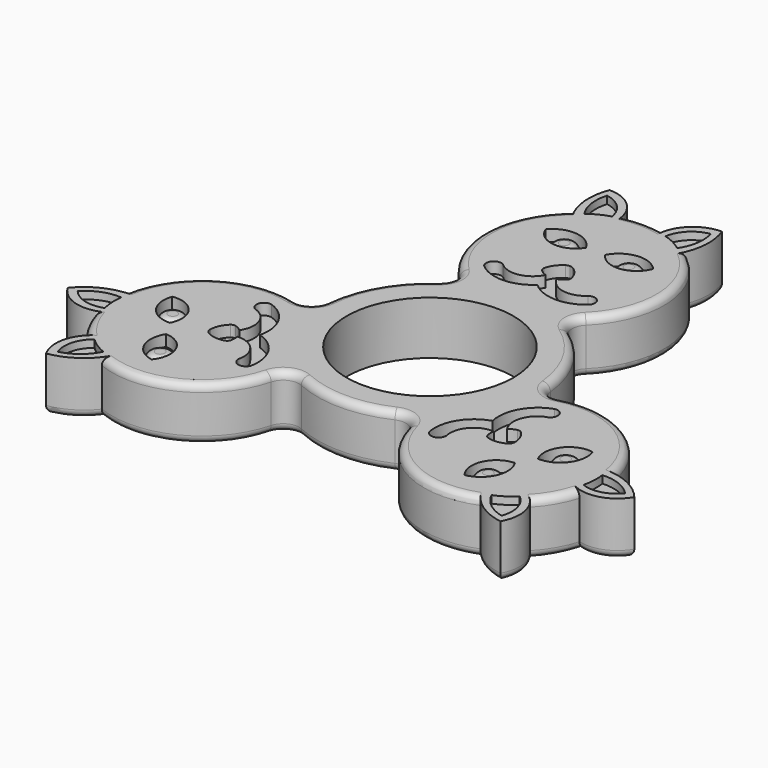
from build123d import *

# Parameters (mm, degrees)
F0_R           = 15
F0_R_2         = 11.125
F1_DEPTH       = 7.1
F3_DEPTH       = 7.1
F5_DEPTH       = 1.5
F6_R           = 1.6130876501
F7_DEPTH       = 1
F8_R           = 0.99999
F10_DEPTH      = 1
F11_R          = 1
F12_T4_ANGLE   = 109.1117538583
F12_S5_R       = 8.0010963912
F12_T6_DEPTH   = 12
F12_T10_ANGLE  = 78.8114219242
F12_S11_R      = 12
F12_T12_DEPTH  = 7
F12_T16_ANGLE  = 134.4694121448
F12_S17_R      = 12
F12_T18_DEPTH  = 7
F12_T22_ANGLE  = 50.774655832
F12_S23_R      = 4.8516880278
F12_T24_DEPTH  = 7
F12_S25_R      = 4.8516880278
F12_T26_DEPTH  = 7
F12_T30_ANGLE  = 134.4694121448
F12_S31_R      = 12
F12_T32_DEPTH  = 7
F12_T36_ANGLE  = 78.8114219242
F12_S37_R      = 12
F12_T38_DEPTH  = 7
F12_T42_ANGLE  = 109.1117538583
F12_S43_R      = 8.0010963912
F12_T44_DEPTH  = 13
F12_T48_ANGLE  = 78.8114219242
F12_S49_R      = 12
F12_T50_DEPTH  = 7
F12_T54_ANGLE  = 134.4694121448
F12_S55_R      = 12
F12_T56_DEPTH  = 7
F12_T60_ANGLE  = 50.774655832
F12_S61_R      = 4.8516880278
F12_T62_DEPTH  = 8
F12_S63_R      = 4.8516880278
F12_T64_DEPTH  = 8
F12_T68_ANGLE  = 134.4694121448
F12_S69_R      = 12
F12_T70_DEPTH  = 7
F12_T74_ANGLE  = 78.8114219242
F12_S75_R      = 12
F12_T76_DEPTH  = 7
F12_T80_ANGLE  = 109.1117538583
F12_S81_R      = 8.0010963912
F12_T82_DEPTH  = 13
F12_T86_ANGLE  = 78.8114219242
F12_S87_R      = 12
F12_T88_DEPTH  = 7
F12_T92_ANGLE  = 134.4694121448
F12_S93_R      = 12
F12_T94_DEPTH  = 7
F12_T98_ANGLE  = 50.774655832
F12_S99_R      = 4.8516880278
F12_T100_DEPTH = 7
F12_S101_R     = 4.8516880278
F12_T102_DEPTH = 7
F12_T106_ANGLE = 134.4694121448
F12_S107_R     = 12
F12_T108_DEPTH = 7
F12_T112_ANGLE = 78.8114219242
F12_S113_R     = 12
F12_T114_DEPTH = 7
F12_T116_ANGLE = 100.004132084
F12_T118_ANGLE = 49.2209251177
F12_T120_ANGLE = 100.004132084
F12_T124_ANGLE = 109.1117538583
F12_S125_R     = 8.0010963912
F12_T126_DEPTH = 13
F12_T128_ANGLE = 100.004132084
F12_T130_ANGLE = 49.2209251177
F12_T132_ANGLE = 100.004132084
F12_T136_ANGLE = 109.1117538583
F12_S137_R     = 8.0010963912
F12_T138_DEPTH = 12
F12_T140_ANGLE = 100.004132084
F12_T142_ANGLE = 49.2209251177
F12_T144_ANGLE = 100.004132084
F12_T148_ANGLE = 109.1117538583
F12_S149_R     = 8.0010963912
F12_T150_DEPTH = 13
F12_T155_ANGLE = 78.8114219242
F12_S156_R     = 12
F12_T157_DEPTH = 7
F12_T160_ANGLE = 109.1117538583
F12_S161_R     = 8.0010963912
F12_T162_DEPTH = 12
F12_T168_ANGLE = 78.8114219242
F12_S169_R     = 12
F12_T170_DEPTH = 7
F12_T173_ANGLE = 109.1117538583
F12_S174_R     = 8.0010963912
F12_T175_DEPTH = 13
F12_T181_ANGLE = 134.4694121448
F12_S182_R     = 12
F12_T183_DEPTH = 7
F12_T186_ANGLE = 50.774655832
F12_S187_R     = 4.8516880278
F12_T188_DEPTH = 7
F12_T194_ANGLE = 134.4694121448
F12_S195_R     = 12
F12_T196_DEPTH = 7
F12_T199_ANGLE = 50.774655832
F12_S200_R     = 4.8516880278
F12_T201_DEPTH = 7
F12_T207_ANGLE = 78.8114219242
F12_S208_R     = 12
F12_T209_DEPTH = 7
F12_T212_ANGLE = 109.1117538583
F12_S213_R     = 8.0010963912
F12_T214_DEPTH = 13
F12_T220_ANGLE = 78.8114219242
F12_S221_R     = 12
F12_T222_DEPTH = 7
F12_T225_ANGLE = 109.1117538583
F12_S226_R     = 8.0010963912
F12_T227_DEPTH = 12
F12_T233_ANGLE = 134.4694121448
F12_S234_R     = 12
F12_T235_DEPTH = 7
F12_T238_ANGLE = 50.774655832
F12_S239_R     = 4.8516880278
F12_T240_DEPTH = 8
F12_T246_ANGLE = 134.4694121448
F12_S247_R     = 12
F12_T248_DEPTH = 7
F12_T251_ANGLE = 50.774655832
F12_S252_R     = 4.8516880278
F12_T253_DEPTH = 8
F12_T259_ANGLE = 78.8114219242
F12_S260_R     = 12
F12_T261_DEPTH = 7
F12_T264_ANGLE = 109.1117538583
F12_S265_R     = 8.0010963912
F12_T266_DEPTH = 13
F12_T272_ANGLE = 78.8114219242
F12_S273_R     = 12
F12_T274_DEPTH = 7
F12_T277_ANGLE = 109.1117538583
F12_S278_R     = 8.0010963912
F12_T279_DEPTH = 13
F12_T285_ANGLE = 134.4694121448
F12_S286_R     = 12
F12_T287_DEPTH = 7
F12_T290_ANGLE = 50.774655832
F12_S291_R     = 4.8516880278
F12_T292_DEPTH = 7
F12_T298_ANGLE = 134.4694121448
F12_S299_R     = 12
F12_T300_DEPTH = 7
F12_T303_ANGLE = 50.774655832
F12_S304_R     = 4.8516880278
F12_T305_DEPTH = 7


# Not quite as in the source:
# - a fillet or chamfer that OpenCascade refuses, or shapes differently, is made with other operations: its cross-section is extruded or revolved along the edge and cut away or added
# - a fillet or chamfer is up to 0.001 mm smaller than in the source, because OpenCascade refuses the exact size


with BuildPart() as f1:
    # F0 (on Top) → F1 (new body)
    with BuildSketch(Plane.XY):
        Circle(F0_R)
        Circle(F0_R_2, mode=Mode.SUBTRACT)
    extrude(amount=F1_DEPTH)

    # F2 (on Top) → F3 (join)
    with BuildSketch(Plane.XY):
        with BuildLine():
            ThreePointArc((-2.7912174802, 35.6708656482), (-4.5237090426, 38.2840211925), (-7.4925607975, 39.2920034192))
            ThreePointArc((-7.4925607975, 39.2920034192), (-8.0154960296, 36.3531541123), (-7.4248709864, 33.4271570919))
            ThreePointArc((-7.4248709864, 33.4271570919), (-11.981393052, 24.6679974054), (-8.4267806253, 15.456618451))
            ThreePointArc((-8.4267806253, 15.456618451), (-7.8041998727, 13.7818905043), (-8.6869847307, 12.2285034362))
            ThreePointArc((-8.6869847307, 12.2285034362), (0, 15), (8.6869847307, 12.2285034362))
            ThreePointArc((8.6869847307, 12.2285034362), (7.8041998727, 13.7818905043), (8.4267806253, 15.456618451))
            ThreePointArc((8.4267806253, 15.456618451), (11.981393052, 24.6679974054), (7.4248709864, 33.4271570919))
            ThreePointArc((7.4248709864, 33.4271570919), (8.0154960296, 36.3531541123), (7.4925607975, 39.2920034192))
            ThreePointArc((7.4925607975, 39.2920034192), (4.5237090426, 38.2840211925), (2.7912174802, 35.6708656482))
            ThreePointArc((2.7912174802, 35.6708656482), (0, 36), (-2.7912174802, 35.6708656482))
        make_face()
        with BuildLine():
            ThreePointArc((-29.4962670862, -20.2526980694), (-30.8930803904, -23.0596575464), (-30.2815927279, -26.1347496997))
            ThreePointArc((-30.2815927279, -26.1347496997), (-27.4750069542, -25.1182002417), (-25.2363317246, -23.14370544))
            ThreePointArc((-25.2363317246, -23.14370544), (-15.3724158876, -22.7101894585), (-9.1724339225, -15.0261153192))
            ThreePointArc((-9.1724339225, -15.0261153192), (-8.0333673526, -13.6495805981), (-6.2467022607, -13.6374011771))
            ThreePointArc((-6.2467022607, -13.6374011771), (-12.9903810568, -7.5), (-14.9336869913, 1.4088977409))
            ThreePointArc((-14.9336869913, 1.4088977409), (-15.8375672253, -0.1323099062), (-17.5992145478, -0.4305031318))
            ThreePointArc((-17.5992145478, -0.4305031318), (-27.3538089396, -1.957807947), (-32.6612027111, -10.2834516518))
            ThreePointArc((-32.6612027111, -10.2834516518), (-35.4905029838, -11.2349538706), (-37.7741535254, -13.1572537196))
            ThreePointArc((-37.7741535254, -13.1572537196), (-35.416789433, -15.224363646), (-32.2874845664, -15.4181675788))
            ThreePointArc((-32.2874845664, -15.4181675788), (-31.1769145362, -18), (-29.4962670862, -20.2526980694))
        make_face()
        with BuildLine():
            ThreePointArc((32.2874845664, -15.4181675788), (35.416789433, -15.224363646), (37.7741535254, -13.1572537196))
            ThreePointArc((37.7741535254, -13.1572537196), (35.4905029838, -11.2349538706), (32.6612027111, -10.2834516518))
            ThreePointArc((32.6612027111, -10.2834516518), (27.3538089396, -1.957807947), (17.5992145478, -0.4305031318))
            ThreePointArc((17.5992145478, -0.4305031318), (15.8375672253, -0.1323099062), (14.9336869913, 1.4088977409))
            ThreePointArc((14.9336869913, 1.4088977409), (12.9903810568, -7.5), (6.2467022607, -13.6374011771))
            ThreePointArc((6.2467022607, -13.6374011771), (8.0333673526, -13.6495805981), (9.1724339225, -15.0261153192))
            ThreePointArc((9.1724339225, -15.0261153192), (15.3724158876, -22.7101894585), (25.2363317246, -23.14370544))
            ThreePointArc((25.2363317246, -23.14370544), (27.4750069542, -25.1182002417), (30.2815927279, -26.1347496997))
            ThreePointArc((30.2815927279, -26.1347496997), (30.8930803904, -23.0596575464), (29.4962670862, -20.2526980694))
            ThreePointArc((29.4962670862, -20.2526980694), (31.1769145362, -18), (32.2874845664, -15.4181675788))
        make_face()
    extrude(amount=F3_DEPTH)

    # F4 (on face) → F5 (cut)
    with BuildSketch(Plane.XY.offset(7.1)):
        with BuildLine():
            ThreePointArc((-7.1594030596, 28.2394494861), (-4.4232053519, 26.0915724177), (-1.2846763711, 27.5915022939))
            ThreePointArc((-1.2846763711, 27.5915022939), (-4.0496666134, 29.478326806), (-7.1594030596, 28.2394494861))
        make_face()
        with BuildLine():
            ThreePointArc((0.5071388441, 23.1854561716), (0.2651917496, 23.3012252013), (0, 23.3414023185))
            ThreePointArc((0, 23.3414023185), (-0.2651917496, 23.3012252013), (-0.5071388441, 23.1854561716))
            ThreePointArc((-0.5071388441, 23.1854561716), (-1.3551723586, 22.3657016302), (-1.826768699, 21.2846117904))
            ThreePointArc((-1.826768699, 21.2846117904), (-1.8109525817, 20.9987396041), (-1.6682691203, 20.7505169494))
            ThreePointArc((-1.6682691203, 20.7505169494), (-1.2370786322, 20.4115554741), (-0.7395183122, 20.180787524))
            ThreePointArc((-0.7395183122, 20.180787524), (-2.9792966503, 18.4746824244), (-5.6797657162, 19.2714687437))
            ThreePointArc((-5.6797657162, 19.2714687437), (-6.9973705426, 19.0919217862), (-6.9920002567, 17.7621508478))
            ThreePointArc((-6.9920002567, 17.7621508478), (-3.4686647794, 16.4959412339), (0, 17.9050346728))
            ThreePointArc((0, 17.9050346728), (3.4686647794, 16.4959412339), (6.9920002567, 17.7621508478))
            ThreePointArc((6.9920002567, 17.7621508478), (6.9973705426, 19.0919217862), (5.6797657162, 19.2714687437))
            ThreePointArc((5.6797657162, 19.2714687437), (2.9792966503, 18.4746824244), (0.7395183122, 20.180787524))
            ThreePointArc((0.7395183122, 20.180787524), (1.2370786322, 20.4115554741), (1.6682691203, 20.7505169494))
            ThreePointArc((1.6682691203, 20.7505169494), (1.8109525817, 20.9987396041), (1.826768699, 21.2846117904))
            ThreePointArc((1.826768699, 21.2846117904), (1.3551723586, 22.3657016302), (0.5071388441, 23.1854561716))
        make_face()
        with BuildLine():
            ThreePointArc((1.2846763711, 27.5915022939), (4.4232053519, 26.0915724177), (7.1594030596, 28.2394494861))
            ThreePointArc((7.1594030596, 28.2394494861), (4.0496666134, 29.478326806), (1.2846763711, 27.5915022939))
        make_face()
        with BuildLine():
            ThreePointArc((-28.0357821737, -7.9194998175), (-27.5538131818, -11.232049239), (-24.5372801007, -12.6831887739))
            ThreePointArc((-24.5372801007, -12.6831887739), (-24.8075672144, -9.2151780079), (-28.0357821737, -7.9194998175))
        make_face()
        with BuildLine():
            ThreePointArc((-18.8784739884, -2.8258255784), (-20.0327745453, -3.4860602435), (-19.5294643584, -4.7169129741))
            ThreePointArc((-19.5294643584, -4.7169129741), (-17.4891926315, -6.6571946277), (-17.8468338203, -9.4499521171))
            ThreePointArc((-17.8468338203, -9.4499521171), (-18.2954648874, -9.1344362151), (-18.80460938, -8.9304950362))
            ThreePointArc((-18.80460938, -8.9304950362), (-19.0909182355, -8.9310388612), (-19.3463988697, -9.060277795))
            ThreePointArc((-19.3463988697, -9.060277795), (-20.0468519645, -10.009237126), (-20.332763465, -11.1535329636))
            ThreePointArc((-20.332763465, -11.1535329636), (-20.3120488384, -11.4209498086), (-20.2142473678, -11.6707011593))
            ThreePointArc((-20.2142473678, -11.6707011593), (-20.0468570888, -11.8802753926), (-19.8256246209, -12.0319232081))
            ThreePointArc((-19.8256246209, -12.0319232081), (-18.6916796059, -12.3564645041), (-17.5196301707, -12.2243339954))
            ThreePointArc((-17.5196301707, -12.2243339954), (-17.2799656538, -12.0677007429), (-17.1363402597, -11.8200219132))
            ThreePointArc((-17.1363402597, -11.8200219132), (-17.0583862552, -11.277119259), (-17.1073155081, -10.7308354069))
            ThreePointArc((-17.1073155081, -10.7308354069), (-14.5098959813, -11.8174877968), (-13.8496986422, -14.5545557696))
            ThreePointArc((-13.8496986422, -14.5545557696), (-13.0354040026, -15.6058615427), (-11.8864737317, -14.9363252695))
            ThreePointArc((-11.8864737317, -14.9363252695), (-12.5515717782, -11.2519224331), (-15.5062148823, -8.9525173364))
            ThreePointArc((-15.5062148823, -8.9525173364), (-16.0202365576, -5.2440188007), (-18.8784739884, -2.8258255784))
        make_face()
        with BuildLine():
            ThreePointArc((-20.8763791141, -20.3199496686), (-20.3843618624, -16.8763944098), (-23.2526037296, -14.90831352))
            ThreePointArc((-23.2526037296, -14.90831352), (-23.5041465684, -18.246277567), (-20.8763791141, -20.3199496686))
        make_face()
        with BuildLine():
            ThreePointArc((20.8763791141, -20.3199496686), (23.5041465684, -18.246277567), (23.2526037296, -14.90831352))
            ThreePointArc((23.2526037296, -14.90831352), (20.3843618624, -16.8763944098), (20.8763791141, -20.3199496686))
        make_face()
        with BuildLine():
            ThreePointArc((11.8864737317, -14.9363252695), (13.0354040026, -15.6058615427), (13.8496986422, -14.5545557696))
            ThreePointArc((13.8496986422, -14.5545557696), (14.5098959813, -11.8174877968), (17.1073155081, -10.7308354069))
            ThreePointArc((17.1073155081, -10.7308354069), (17.0583862552, -11.277119259), (17.1363402597, -11.8200219132))
            ThreePointArc((17.1363402597, -11.8200219132), (17.2799656538, -12.0677007429), (17.5196301707, -12.2243339954))
            ThreePointArc((17.5196301707, -12.2243339954), (18.6916796059, -12.3564645041), (19.8256246209, -12.0319232081))
            ThreePointArc((19.8256246209, -12.0319232081), (20.0468570888, -11.8802753926), (20.2142473678, -11.6707011593))
            ThreePointArc((20.2142473678, -11.6707011593), (20.3120488384, -11.4209498086), (20.332763465, -11.1535329636))
            ThreePointArc((20.332763465, -11.1535329636), (20.0468519645, -10.009237126), (19.3463988697, -9.060277795))
            ThreePointArc((19.3463988697, -9.060277795), (19.0909182355, -8.9310388612), (18.80460938, -8.9304950362))
            ThreePointArc((18.80460938, -8.9304950362), (18.2954648874, -9.1344362151), (17.8468338203, -9.4499521171))
            ThreePointArc((17.8468338203, -9.4499521171), (17.4891926315, -6.6571946277), (19.5294643584, -4.7169129741))
            ThreePointArc((19.5294643584, -4.7169129741), (20.0327745453, -3.4860602435), (18.8784739884, -2.8258255784))
            ThreePointArc((18.8784739884, -2.8258255784), (16.0202365576, -5.2440188007), (15.5062148823, -8.9525173364))
            ThreePointArc((15.5062148823, -8.9525173364), (12.5515717782, -11.2519224331), (11.8864737317, -14.9363252695))
        make_face()
        with BuildLine():
            ThreePointArc((28.0357821737, -7.9194998175), (24.8075672144, -9.2151780079), (24.5372801007, -12.6831887739))
            ThreePointArc((24.5372801007, -12.6831887739), (27.5538131818, -11.232049239), (28.0357821737, -7.9194998175))
        make_face()
    extrude(amount=-F5_DEPTH, mode=Mode.SUBTRACT)

    # F6 (on face) → F7 (join)
    with BuildSketch(Plane.XY.offset(5.6)):
        with Locations((-4.3190591969, 27.7605038136)):
            Circle(F6_R)
        with Locations((4.3190591969, 27.7605038136)):
            Circle(F6_R)
        with Locations((-21.881771926, -17.6206668917)):
            Circle(F6_R)
        with Locations((-26.2008311229, -10.1398369219)):
            Circle(F6_R)
        with Locations((26.2008311229, -10.1398369219)):
            Circle(F6_R)
        with Locations((21.881771926, -17.6206668917)):
            Circle(F6_R)
    extrude(amount=F7_DEPTH)

    # F8 (radius 1 in the source; OpenCascade refuses exactly that, so slightly less here)
    f8_edges = [f1.edges().sort_by_distance(p)[0] for p in [
        (2.705972, 27.760504, 6.6),
        (-5.932147, 27.760504, 6.6),
        (-27.813919, -10.139837, 6.6),
        (-23.49486, -17.620667, 6.6),
        (20.268684, -17.620667, 6.6),
        (24.587743, -10.139837, 6.6),
    ]]
    fillet(f8_edges, radius=F8_R)

    # F9 (on face) → F10 (cut)
    with BuildSketch(Plane.XY.offset(7.1)):
        with BuildLine():
            ThreePointArc((-3.5642137217, 34.7998360329), (-4.6967498159, 37.0173790956), (-6.9121797569, 38.1540432572))
            ThreePointArc((-6.9121797569, 38.1540432572), (-7.0803269374, 35.7276423867), (-6.1938797928, 33.4627127811))
            ThreePointArc((-6.1938797928, 33.4627127811), (-4.9436251849, 34.2582781816), (-3.5642137217, 34.7998360329))
        make_face()
        with BuildLine():
            ThreePointArc((6.9121797569, 38.1540432572), (4.6967498159, 37.0173790956), (3.5642137217, 34.7998360329))
            ThreePointArc((3.5642137217, 34.7998360329), (4.9436251849, 34.2582781816), (6.1938797928, 33.4627127811))
            ThreePointArc((6.1938797928, 33.4627127811), (7.0803269374, 35.7276423867), (6.9121797569, 38.1540432572))
        make_face()
        with BuildLine():
            ThreePointArc((-32.0764992444, -11.367299142), (-34.4812093929, -11.7320781985), (-36.4984605963, -13.0908983636))
            ThreePointArc((-36.4984605963, -13.0908983636), (-34.4063655863, -14.441184892), (-31.9196489129, -14.3132183889))
            ThreePointArc((-31.9196489129, -14.3132183889), (-32.1403517876, -12.8478340939), (-32.0764992444, -11.367299142))
        make_face()
        with BuildLine():
            ThreePointArc((-25.8826194516, -22.0954136391), (-27.1967266027, -21.4104440877), (-28.3554351912, -20.486617644))
            ThreePointArc((-28.3554351912, -20.486617644), (-29.7096157704, -22.5761942036), (-29.5862808394, -25.0631448936))
            ThreePointArc((-29.5862808394, -25.0631448936), (-27.4008824556, -23.9955641882), (-25.8826194516, -22.0954136391))
        make_face()
        with BuildLine():
            ThreePointArc((25.8826194516, -22.0954136391), (27.4008824556, -23.9955641882), (29.5862808394, -25.0631448936))
            ThreePointArc((29.5862808394, -25.0631448936), (29.7096157704, -22.5761942036), (28.3554351912, -20.486617644))
            ThreePointArc((28.3554351912, -20.486617644), (27.1967266027, -21.4104440877), (25.8826194516, -22.0954136391))
        make_face()
        with BuildLine():
            ThreePointArc((32.0764992444, -11.367299142), (32.1403517876, -12.8478340939), (31.9196489129, -14.3132183889))
            ThreePointArc((31.9196489129, -14.3132183889), (34.4063655863, -14.441184892), (36.4984605963, -13.0908983636))
            ThreePointArc((36.4984605963, -13.0908983636), (34.4812093929, -11.7320781985), (32.0764992444, -11.367299142))
        make_face()
    extrude(amount=-F10_DEPTH, mode=Mode.SUBTRACT)

    # F11
    f11_edges = [f1.edges().sort_by_distance(p)[0] for p in [
        (-11.981393, 24.667997, 7.1),
        (0, 36, 7.1),
        (11.981393, 24.667997, 7.1),
        (31.176915, -18, 7.1),
        (15.372416, -22.710189, 7.1),
        (-31.176915, -18, 7.1),
    ]]
    fillet(f11_edges, radius=F11_R)

    # F12: fillet of radius 1 on 18 edges, made by hand


with BuildPart() as f12_tool2:
    # F12_s3 → F12_t4 (revolve)
    with BuildSketch(Plane(origin=(-0.6891266462, -10.6045494997, 0), x_dir=(0, 0, 1), z_dir=(-0.0648472783, -0.9978952002, 0))):
        with BuildLine():
            ThreePointArc((0, -32.5190295872), (0.2928932188, -33.2261363683), (1, -33.5190295872))
            Line((1, -33.5190295872), (0, -33.5190295872))
            Line((0, -33.5190295872), (0, -32.5190295872))
        make_face()
    revolve(axis=Axis((20.7846096908, -12, 0), (0, 0, 1)), revolution_arc=F12_T4_ANGLE)

    # F12_s5 → F12_t6 (cut, symmetric)
    with BuildSketch(Plane.XY.offset(0.9)):
        with Locations((31.570189518, -18.2098148579)):
            Circle(F12_S5_R)
    extrude(amount=F12_T6_DEPTH, both=True, mode=Mode.SUBTRACT)


with BuildPart() as f1_1:
    add(f1.part)

    # F12_t1: cut F12_tool2
    add(f12_tool2.part, mode=Mode.SUBTRACT)


with BuildPart() as f12_tool8:
    # F12_s9 → F12_t10 (revolve)
    with BuildSketch(Plane(origin=(17.959437211, 21.352490272, 0), x_dir=(0, 0, 1), z_dir=(-0.6436825265, -0.7652926271, 0))):
        with BuildLine():
            ThreePointArc((1, 15.4468032505), (0.2928932188, 15.7396964693), (0, 16.4468032505))
            Line((0, 16.4468032505), (0, 15.4468032505))
            Line((0, 15.4468032505), (1, 15.4468032505))
        make_face()
    revolve(axis=Axis((0.0149324938, 36.4454935538, 0), (0, 0, 1)), revolution_arc=F12_T10_ANGLE)

    # F12_s11 → F12_t12 (cut, symmetric)
    with BuildSketch(Plane.XY.offset(0.5)):
        with Locations((0, 24)):
            Circle(F12_S11_R)
    extrude(amount=F12_T12_DEPTH, both=True, mode=Mode.SUBTRACT)


with BuildPart() as f1_2:
    add(f1_1.part)

    # F12_t7: cut F12_tool8
    add(f12_tool8.part, mode=Mode.SUBTRACT)


with BuildPart() as f12_tool14:
    # F12_s15 → F12_t16 (revolve)
    with BuildSketch(Plane(origin=(-9.1457575859, 5.2018480745, 0), x_dir=(0, 0, 1), z_dir=(0.8692362368, -0.4943969707, 0))):
        with BuildLine():
            ThreePointArc((1, -38.4886594065), (0.2928932188, -38.1957661877), (0, -37.4886594065))
            Line((0, -37.4886594065), (0, -38.4886594065))
            Line((0, -38.4886594065), (1, -38.4886594065))
        make_face()
    revolve(axis=Axis((7.4842591659, 34.4403224938, 0), (0, 0, 1)), revolution_arc=F12_T16_ANGLE)

    # F12_s17 → F12_t18 (cut, symmetric)
    with BuildSketch(Plane.XY.offset(0.5)):
        with Locations((0, 24)):
            Circle(F12_S17_R)
    extrude(amount=F12_T18_DEPTH, both=True, mode=Mode.SUBTRACT)


with BuildPart() as f1_3:
    add(f1_2.part)

    # F12_t13: cut F12_tool14
    add(f12_tool14.part, mode=Mode.SUBTRACT)


with BuildPart() as f12_tool20:
    # F12_s21 → F12_t22 (revolve)
    with BuildSketch(Plane(origin=(-9.2959780989, 4.4115356505, 0), x_dir=(0, 0, 1), z_dir=(0.9034301382, -0.4287353326, 0))):
        with BuildLine():
            ThreePointArc((0, -32.6823233162), (0.2928932188, -33.3894300974), (1, -33.6823233162))
            Line((1, -33.6823233162), (0, -33.6823233162))
            Line((0, -33.6823233162), (0, -32.6823233162))
        make_face()
    revolve(axis=Axis((0, 24, 0), (0, 0, 1)), revolution_arc=F12_T22_ANGLE)

    # F12_s23 → F12_t24 (cut, symmetric)
    with BuildSketch(Plane.XY.offset(0.9)):
        with Locations((-7.4842591659, 34.4403224938)):
            Circle(F12_S23_R)
    extrude(amount=F12_T24_DEPTH, both=True, mode=Mode.SUBTRACT)

    # F12_s25 → F12_t26 (cut, symmetric)
    with BuildSketch(Plane.XY.offset(0.9)):
        with Locations((7.4842591659, 34.4403224938)):
            Circle(F12_S25_R)
    extrude(amount=F12_T26_DEPTH, both=True, mode=Mode.SUBTRACT)


with BuildPart() as f1_4:
    add(f1_3.part)

    # F12_t19: cut F12_tool20
    add(f12_tool20.part, mode=Mode.SUBTRACT)


with BuildPart() as f12_tool28:
    # F12_s29 → F12_t30 (revolve)
    with BuildSketch(Plane(origin=(8.0354392986, 30.3284166009, 0), x_dir=(0, 0, 1), z_dir=(-0.2561108532, -0.9666474181, 0))):
        with BuildLine():
            ThreePointArc((1, 11.2034921488), (0.2928932188, 11.4963853676), (0, 12.2034921488))
            Line((0, 12.2034921488), (0, 11.2034921488))
            Line((0, 11.2034921488), (1, 11.2034921488))
        make_face()
    revolve(axis=Axis((-7.4842591659, 34.4403224938, 0), (0, 0, 1)), revolution_arc=F12_T30_ANGLE)

    # F12_s31 → F12_t32 (cut, symmetric)
    with BuildSketch(Plane.XY.offset(0.5)):
        with Locations((0, 24)):
            Circle(F12_S31_R)
    extrude(amount=F12_T32_DEPTH, both=True, mode=Mode.SUBTRACT)


with BuildPart() as f1_5:
    add(f1_4.part)

    # F12_t27: cut F12_tool28
    add(f12_tool28.part, mode=Mode.SUBTRACT)


with BuildPart() as f12_tool34:
    # F12_s35 → F12_t36 (revolve)
    with BuildSketch(Plane(origin=(17.7841822398, 22.1630259504, 0), x_dir=(0, 0, 1), z_dir=(0.6258479846, 0.7799450623, 0))):
        with BuildLine():
            ThreePointArc((1, -30.8220816054), (0.2928932188, -30.5291883866), (0, -29.8220816054))
            Line((0, -29.8220816054), (0, -30.8220816054))
            Line((0, -30.8220816054), (1, -30.8220816054))
        make_face()
    revolve(axis=Axis((-0.0149324938, 36.4454935538, 0), (0, 0, 1)), revolution_arc=F12_T36_ANGLE)

    # F12_s37 → F12_t38 (cut, symmetric)
    with BuildSketch(Plane.XY.offset(0.5)):
        with Locations((0, 24)):
            Circle(F12_S37_R)
    extrude(amount=F12_T38_DEPTH, both=True, mode=Mode.SUBTRACT)


with BuildPart() as f1_6:
    add(f1_5.part)

    # F12_t33: cut F12_tool34
    add(f12_tool34.part, mode=Mode.SUBTRACT)


with BuildPart() as f12_tool40:
    # F12_s41 → F12_t42 (revolve)
    with BuildSketch(Plane(origin=(9.5283725856, 4.7054735678, 0), x_dir=(0, 0, 1), z_dir=(0.8966262328, 0.4427882097, 0))):
        with BuildLine():
            ThreePointArc((1, -33.5190295872), (0.2928932188, -33.2261363683), (0, -32.5190295872))
            Line((0, -32.5190295872), (0, -33.5190295872))
            Line((0, -33.5190295872), (1, -33.5190295872))
        make_face()
    revolve(axis=Axis((0, 24, 0), (0, 0, 1)), revolution_arc=F12_T42_ANGLE)

    # F12_s43 → F12_t44 (cut, symmetric)
    with BuildSketch(Plane.XY.offset(0.5)):
        with Locations((-0.0149324938, 36.4454935538)):
            Circle(F12_S43_R)
    extrude(amount=F12_T44_DEPTH, both=True, mode=Mode.SUBTRACT)


with BuildPart() as f1_7:
    add(f1_6.part)

    # F12_t39: cut F12_tool40
    add(f12_tool40.part, mode=Mode.SUBTRACT)


with BuildPart() as f12_tool46:
    # F12_s47 → F12_t48 (revolve)
    with BuildSketch(Plane(origin=(-27.4715176151, 4.8770837264, 0), x_dir=(0, 0, 1), z_dir=(0.9846041196, -0.1747991063, 0))):
        with BuildLine():
            ThreePointArc((1, 15.4468032505), (0.2928932188, 15.7396964693), (0, 16.4468032505))
            Line((0, 16.4468032505), (0, 15.4468032505))
            Line((0, 15.4468032505), (1, 15.4468032505))
        make_face()
    revolve(axis=Axis((-31.570189518, -18.2098148579, 0), (0, 0, 1)), revolution_arc=F12_T48_ANGLE)

    # F12_s49 → F12_t50 (cut, symmetric)
    with BuildSketch(Plane.XY.offset(0.5)):
        with Locations((-20.7846096908, -12)):
            Circle(F12_S49_R)
    extrude(amount=F12_T50_DEPTH, both=True, mode=Mode.SUBTRACT)


with BuildPart() as f1_8:
    add(f1_7.part)

    # F12_t45: cut F12_tool46
    add(f12_tool46.part, mode=Mode.SUBTRACT)


with BuildPart() as f12_tool52:
    # F12_s53 → F12_t54 (revolve)
    with BuildSketch(Plane(origin=(0.0679462137, -10.5213824435, 0), x_dir=(0, 0, 1), z_dir=(-0.0064577823, 0.9999791483, 0))):
        with BuildLine():
            ThreePointArc((1, -38.4886594065), (0.2928932188, -38.1957661877), (0, -37.4886594065))
            Line((0, -37.4886594065), (0, -38.4886594065))
            Line((0, -38.4886594065), (1, -38.4886594065))
        make_face()
    revolve(axis=Axis((-33.5683237772, -10.7386026807, 0), (0, 0, 1)), revolution_arc=F12_T54_ANGLE)

    # F12_s55 → F12_t56 (cut, symmetric)
    with BuildSketch(Plane.XY.offset(0.5)):
        with Locations((-20.7846096908, -12)):
            Circle(F12_S55_R)
    extrude(amount=F12_T56_DEPTH, both=True, mode=Mode.SUBTRACT)


with BuildPart() as f1_9:
    add(f1_8.part)

    # F12_t51: cut F12_tool52
    add(f12_tool52.part, mode=Mode.SUBTRACT)


with BuildPart() as f12_tool58:
    # F12_s59 → F12_t60 (revolve)
    with BuildSketch(Plane(origin=(0.8274871065, -10.2563210119, 0), x_dir=(0, 0, 1), z_dir=(-0.0804193795, 0.9967611165, 0))):
        with BuildLine():
            ThreePointArc((0, -32.6823233162), (0.2928932188, -33.3894300974), (1, -33.6823233162))
            Line((1, -33.6823233162), (0, -33.6823233162))
            Line((0, -33.6823233162), (0, -32.6823233162))
        make_face()
    revolve(axis=Axis((-20.7846096908, -12, 0), (0, 0, 1)), revolution_arc=F12_T60_ANGLE)

    # F12_s61 → F12_t62 (cut, symmetric)
    with BuildSketch(Plane.XY.offset(0.9)):
        with Locations((-33.5683237772, -10.7386026807)):
            Circle(F12_S61_R)
    extrude(amount=F12_T62_DEPTH, both=True, mode=Mode.SUBTRACT)

    # F12_s63 → F12_t64 (cut, symmetric)
    with BuildSketch(Plane.XY.offset(0.9)):
        with Locations((-26.0840646112, -23.7017198131)):
            Circle(F12_S63_R)
    extrude(amount=F12_T64_DEPTH, both=True, mode=Mode.SUBTRACT)


with BuildPart() as f1_10:
    add(f1_9.part)

    # F12_t57: cut F12_tool58
    add(f12_tool58.part, mode=Mode.SUBTRACT)


with BuildPart() as f12_tool66:
    # F12_s67 → F12_t68 (revolve)
    with BuildSketch(Plane(origin=(-30.2828988822, -8.2053137373, 0), x_dir=(0, 0, 1), z_dir=(0.9651966471, 0.261525204, 0))):
        with BuildLine():
            ThreePointArc((1, 11.2034921488), (0.2928932188, 11.4963853676), (0, 12.2034921488))
            Line((0, 12.2034921488), (0, 11.2034921488))
            Line((0, 11.2034921488), (1, 11.2034921488))
        make_face()
    revolve(axis=Axis((-26.0840646112, -23.7017198131, 0), (0, 0, 1)), revolution_arc=F12_T68_ANGLE)

    # F12_s69 → F12_t70 (cut, symmetric)
    with BuildSketch(Plane.XY.offset(0.5)):
        with Locations((-20.7846096908, -12)):
            Circle(F12_S69_R)
    extrude(amount=F12_T70_DEPTH, both=True, mode=Mode.SUBTRACT)


with BuildPart() as f1_11:
    add(f1_10.part)

    # F12_t65: cut F12_tool66
    add(f12_tool66.part, mode=Mode.SUBTRACT)


with BuildPart() as f12_tool72:
    # F12_s73 → F12_t74 (revolve)
    with BuildSketch(Plane(origin=(-28.0858346177, 4.32004063, 0), x_dir=(0, 0, 1), z_dir=(-0.9883762298, 0.1520277225, 0))):
        with BuildLine():
            ThreePointArc((1, -30.8220816054), (0.2928932188, -30.5291883866), (0, -29.8220816054))
            Line((0, -29.8220816054), (0, -30.8220816054))
            Line((0, -30.8220816054), (1, -30.8220816054))
        make_face()
    revolve(axis=Axis((-31.5552570241, -18.2356786959, 0), (0, 0, 1)), revolution_arc=F12_T74_ANGLE)

    # F12_s75 → F12_t76 (cut, symmetric)
    with BuildSketch(Plane.XY.offset(0.5)):
        with Locations((-20.7846096908, -12)):
            Circle(F12_S75_R)
    extrude(amount=F12_T76_DEPTH, both=True, mode=Mode.SUBTRACT)


with BuildPart() as f1_12:
    add(f1_11.part)

    # F12_t71: cut F12_tool72
    add(f12_tool72.part, mode=Mode.SUBTRACT)


with BuildPart() as f12_tool78:
    # F12_s79 → F12_t80 (revolve)
    with BuildSketch(Plane(origin=(-8.8392459393, 5.8990759319, 0), x_dir=(0, 0, 1), z_dir=(-0.8317789545, 0.5551069904, 0))):
        with BuildLine():
            ThreePointArc((0, -32.5190295872), (0.2928932188, -33.2261363683), (1, -33.5190295872))
            Line((1, -33.5190295872), (0, -33.5190295872))
            Line((0, -33.5190295872), (0, -32.5190295872))
        make_face()
    revolve(axis=Axis((-20.7846096908, -12, 0), (0, 0, 1)), revolution_arc=F12_T80_ANGLE)

    # F12_s81 → F12_t82 (cut, symmetric)
    with BuildSketch(Plane.XY.offset(0.9)):
        with Locations((-31.5552570241, -18.2356786959)):
            Circle(F12_S81_R)
    extrude(amount=F12_T82_DEPTH, both=True, mode=Mode.SUBTRACT)


with BuildPart() as f1_13:
    add(f1_12.part)

    # F12_t77: cut F12_tool78
    add(f12_tool78.part, mode=Mode.SUBTRACT)


with BuildPart() as f12_tool84:
    # F12_s85 → F12_t86 (revolve)
    with BuildSketch(Plane(origin=(9.5120804041, -26.2295739984, 0), x_dir=(0, 0, 1), z_dir=(-0.3409215932, 0.9400917335, 0))):
        with BuildLine():
            ThreePointArc((1, 15.4468032505), (0.2928932188, 15.7396964693), (0, 16.4468032505))
            Line((0, 16.4468032505), (0, 15.4468032505))
            Line((0, 15.4468032505), (1, 15.4468032505))
        make_face()
    revolve(axis=Axis((31.5552570241, -18.2356786959, 0), (0, 0, 1)), revolution_arc=F12_T86_ANGLE)

    # F12_s87 → F12_t88 (cut, symmetric)
    with BuildSketch(Plane.XY.offset(0.5)):
        with Locations((20.7846096908, -12)):
            Circle(F12_S87_R)
    extrude(amount=F12_T88_DEPTH, both=True, mode=Mode.SUBTRACT)


with BuildPart() as f1_14:
    add(f1_13.part)

    # F12_t83: cut F12_tool84
    add(f12_tool84.part, mode=Mode.SUBTRACT)


with BuildPart() as f12_tool90:
    # F12_s91 → F12_t92 (revolve)
    with BuildSketch(Plane(origin=(9.0778113721, 5.3195343689, 0), x_dir=(0, 0, 1), z_dir=(-0.8627784546, -0.5055821776, 0))):
        with BuildLine():
            ThreePointArc((1, -38.4886594065), (0.2928932188, -38.1957661877), (0, -37.4886594065))
            Line((0, -37.4886594065), (0, -38.4886594065))
            Line((0, -38.4886594065), (1, -38.4886594065))
        make_face()
    revolve(axis=Axis((26.0840646112, -23.7017198131, 0), (0, 0, 1)), revolution_arc=F12_T92_ANGLE)

    # F12_s93 → F12_t94 (cut, symmetric)
    with BuildSketch(Plane.XY.offset(0.5)):
        with Locations((20.7846096908, -12)):
            Circle(F12_S93_R)
    extrude(amount=F12_T94_DEPTH, both=True, mode=Mode.SUBTRACT)


with BuildPart() as f1_15:
    add(f1_14.part)

    # F12_t89: cut F12_tool90
    add(f12_tool90.part, mode=Mode.SUBTRACT)


with BuildPart() as f12_tool96:
    # F12_s97 → F12_t98 (revolve)
    with BuildSketch(Plane(origin=(8.4684909925, 5.8447853615, 0), x_dir=(0, 0, 1), z_dir=(-0.8230107586, -0.5680257839, 0))):
        with BuildLine():
            ThreePointArc((0, -32.6823233162), (0.2928932188, -33.3894300974), (1, -33.6823233162))
            Line((1, -33.6823233162), (0, -33.6823233162))
            Line((0, -33.6823233162), (0, -32.6823233162))
        make_face()
    revolve(axis=Axis((20.7846096908, -12, 0), (0, 0, 1)), revolution_arc=F12_T98_ANGLE)

    # F12_s99 → F12_t100 (cut, symmetric)
    with BuildSketch(Plane.XY.offset(0.9)):
        with Locations((33.5683237772, -10.7386026807)):
            Circle(F12_S99_R)
    extrude(amount=F12_T100_DEPTH, both=True, mode=Mode.SUBTRACT)

    # F12_s101 → F12_t102 (cut, symmetric)
    with BuildSketch(Plane.XY.offset(0.9)):
        with Locations((26.0840646112, -23.7017198131)):
            Circle(F12_S101_R)
    extrude(amount=F12_T102_DEPTH, both=True, mode=Mode.SUBTRACT)


with BuildPart() as f1_16:
    add(f1_15.part)

    # F12_t95: cut F12_tool96
    add(f12_tool96.part, mode=Mode.SUBTRACT)


with BuildPart() as f12_tool104:
    # F12_s105 → F12_t106 (revolve)
    with BuildSketch(Plane(origin=(22.2474595837, -22.1231028636, 0), x_dir=(0, 0, 1), z_dir=(-0.709085794, 0.7051222141, 0))):
        with BuildLine():
            ThreePointArc((1, 11.2034921488), (0.2928932188, 11.4963853676), (0, 12.2034921488))
            Line((0, 12.2034921488), (0, 11.2034921488))
            Line((0, 11.2034921488), (1, 11.2034921488))
        make_face()
    revolve(axis=Axis((33.5683237772, -10.7386026807, 0), (0, 0, 1)), revolution_arc=F12_T106_ANGLE)

    # F12_s107 → F12_t108 (cut, symmetric)
    with BuildSketch(Plane.XY.offset(0.5)):
        with Locations((20.7846096908, -12)):
            Circle(F12_S107_R)
    extrude(amount=F12_T108_DEPTH, both=True, mode=Mode.SUBTRACT)


with BuildPart() as f1_17:
    add(f1_16.part)

    # F12_t103: cut F12_tool104
    add(f12_tool104.part, mode=Mode.SUBTRACT)


with BuildPart() as f12_tool110:
    # F12_s111 → F12_t112 (revolve)
    with BuildSketch(Plane(origin=(10.3016523779, -26.4830665804, 0), x_dir=(0, 0, 1), z_dir=(0.3625282452, -0.9319727847, 0))):
        with BuildLine():
            ThreePointArc((1, -30.8220816054), (0.2928932188, -30.5291883866), (0, -29.8220816054))
            Line((0, -29.8220816054), (0, -30.8220816054))
            Line((0, -30.8220816054), (1, -30.8220816054))
        make_face()
    revolve(axis=Axis((31.570189518, -18.2098148579, 0), (0, 0, 1)), revolution_arc=F12_T112_ANGLE)

    # F12_s113 → F12_t114 (cut, symmetric)
    with BuildSketch(Plane.XY.offset(0.5)):
        with Locations((20.7846096908, -12)):
            Circle(F12_S113_R)
    extrude(amount=F12_T114_DEPTH, both=True, mode=Mode.SUBTRACT)


with BuildPart() as f1_18:
    add(f1_17.part)

    # F12_t109: cut F12_tool110
    add(f12_tool110.part, mode=Mode.SUBTRACT)

    # F12_s115 → F12_t116 (revolve, cut)
    with BuildSketch(Plane(origin=(-4.2500683236, -16.3088762972, 0), x_dir=(0, 0, 1), z_dir=(-0.2521762766, -0.967681314, 0))):
        with BuildLine():
            ThreePointArc((0, 6.0867630981), (0.2928932188, 5.3796563169), (1, 5.0867630981))
            Line((1, 5.0867630981), (0, 5.0867630981))
            Line((0, 5.0867630981), (0, 6.0867630981))
        make_face()
    revolve(axis=Axis((-7.126975995, -15.5591585397, 0), (0, 0, -1)), revolution_arc=F12_T116_ANGLE, mode=Mode.SUBTRACT)

    # F12_s117 → F12_t118 (revolve, cut)
    with BuildSketch(Plane(origin=(0, 0, 0), x_dir=(0, 0, 1), z_dir=(-0.9091600785, 0.4164468174, 0))):
        with BuildLine():
            ThreePointArc((0, -14), (0.2928932188, -14.7071067812), (1, -15))
            Line((1, -15), (0, -15))
            Line((0, -15), (0, -14))
        make_face()
    revolve(axis=Axis((0, 0, 0), (0, 0, 1)), revolution_arc=F12_T118_ANGLE, mode=Mode.SUBTRACT)

    # F12_s119 → F12_t120 (revolve, cut)
    with BuildSketch(Plane(origin=(0, 0, 0), x_dir=(0, 0, 1), z_dir=(-0.9091600785, -0.4164468174, 0))):
        with BuildLine():
            ThreePointArc((0, -14), (0.2928932188, -14.7071067812), (1, -15))
            Line((1, -15), (0, -15))
            Line((0, -15), (0, -14))
        make_face()
    revolve(axis=Axis((7.126975995, -15.5591585397, 0), (0, 0, -1)), revolution_arc=F12_T120_ANGLE, mode=Mode.SUBTRACT)


with BuildPart() as f12_tool122:
    # F12_s123 → F12_t124 (revolve)
    with BuildSketch(Plane(origin=(4.2500683236, -16.3088762972, 0), x_dir=(0, 0, 1), z_dir=(-0.2521762766, 0.967681314, 0))):
        with BuildLine():
            ThreePointArc((0, 6.0867630981), (0.2928932188, 5.3796563169), (1, 5.0867630981))
            Line((1, 5.0867630981), (0, 5.0867630981))
            Line((0, 5.0867630981), (0, 6.0867630981))
        make_face()
    revolve(axis=Axis((20.7846096908, -12, 0), (0, 0, 1)), revolution_arc=F12_T124_ANGLE)

    # F12_s125 → F12_t126 (cut, symmetric)
    with BuildSketch(Plane.XY.offset(0.9)):
        with Locations((31.5552570241, -18.2356786959)):
            Circle(F12_S125_R)
    extrude(amount=F12_T126_DEPTH, both=True, mode=Mode.SUBTRACT)


with BuildPart() as f1_19:
    add(f1_18.part)

    # F12_t121: cut F12_tool122
    add(f12_tool122.part, mode=Mode.SUBTRACT)

    # F12_s127 → F12_t128 (revolve, cut)
    with BuildSketch(Plane(origin=(-11.9988670187, 11.8351052846, 0), x_dir=(0, 0, 1), z_dir=(-0.7119484624, 0.7022317188, 0))):
        with BuildLine():
            ThreePointArc((0, 6.0867630981), (0.2928932188, 5.3796563169), (1, 5.0867630981))
            Line((1, 5.0867630981), (0, 5.0867630981))
            Line((0, 5.0867630981), (0, 6.0867630981))
        make_face()
    revolve(axis=Axis((-9.9111385594, 13.9517215337, 0), (0, 0, -1)), revolution_arc=F12_T128_ANGLE, mode=Mode.SUBTRACT)

    # F12_s129 → F12_t130 (revolve, cut)
    with BuildSketch(Plane(origin=(0, 0, 0), x_dir=(0, 0, 1), z_dir=(0.8152335624, 0.5791323154, 0))):
        with BuildLine():
            ThreePointArc((0, -14), (0.2928932188, -14.7071067812), (1, -15))
            Line((1, -15), (0, -15))
            Line((0, -15), (0, -14))
        make_face()
    revolve(axis=Axis((0, 0, 0), (0, 0, 1)), revolution_arc=F12_T130_ANGLE, mode=Mode.SUBTRACT)

    # F12_s131 → F12_t132 (revolve, cut)
    with BuildSketch(Plane(origin=(0, 0, 0), x_dir=(0, 0, 1), z_dir=(0.0939265161, 0.9955791328, 0))):
        with BuildLine():
            ThreePointArc((0, -14), (0.2928932188, -14.7071067812), (1, -15))
            Line((1, -15), (0, -15))
            Line((0, -15), (0, -14))
        make_face()
    revolve(axis=Axis((-17.0381145544, 1.607437006, 0), (0, 0, -1)), revolution_arc=F12_T132_ANGLE, mode=Mode.SUBTRACT)


with BuildPart() as f12_tool134:
    # F12_s135 → F12_t136 (revolve)
    with BuildSketch(Plane(origin=(-16.2489353423, 4.4737710125, 0), x_dir=(0, 0, 1), z_dir=(0.964124739, -0.2654495953, 0))):
        with BuildLine():
            ThreePointArc((0, 6.0867630981), (0.2928932188, 5.3796563169), (1, 5.0867630981))
            Line((1, 5.0867630981), (0, 5.0867630981))
            Line((0, 5.0867630981), (0, 6.0867630981))
        make_face()
    revolve(axis=Axis((-20.7846096908, -12, 0), (0, 0, 1)), revolution_arc=F12_T136_ANGLE)

    # F12_s137 → F12_t138 (cut, symmetric)
    with BuildSketch(Plane.XY.offset(0.9)):
        with Locations((-31.570189518, -18.2098148579)):
            Circle(F12_S137_R)
    extrude(amount=F12_T138_DEPTH, both=True, mode=Mode.SUBTRACT)


with BuildPart() as f1_20:
    add(f1_19.part)

    # F12_t133: cut F12_tool134
    add(f12_tool134.part, mode=Mode.SUBTRACT)

    # F12_s139 → F12_t140 (revolve, cut)
    with BuildSketch(Plane(origin=(16.2489353423, 4.4737710125, 0), x_dir=(0, 0, 1), z_dir=(0.964124739, 0.2654495953, 0))):
        with BuildLine():
            ThreePointArc((0, 6.0867630981), (0.2928932188, 5.3796563169), (1, 5.0867630981))
            Line((1, 5.0867630981), (0, 5.0867630981))
            Line((0, 5.0867630981), (0, 6.0867630981))
        make_face()
    revolve(axis=Axis((17.0381145544, 1.607437006, 0), (0, 0, -1)), revolution_arc=F12_T140_ANGLE, mode=Mode.SUBTRACT)

    # F12_s141 → F12_t142 (revolve, cut)
    with BuildSketch(Plane(origin=(0, 0, 0), x_dir=(0, 0, 1), z_dir=(0.0939265161, -0.9955791328, 0))):
        with BuildLine():
            ThreePointArc((0, -14), (0.2928932188, -14.7071067812), (1, -15))
            Line((1, -15), (0, -15))
            Line((0, -15), (0, -14))
        make_face()
    revolve(axis=Axis((0, 0, 0), (0, 0, 1)), revolution_arc=F12_T142_ANGLE, mode=Mode.SUBTRACT)

    # F12_s143 → F12_t144 (revolve, cut)
    with BuildSketch(Plane(origin=(0, 0, 0), x_dir=(0, 0, 1), z_dir=(0.8152335624, -0.5791323154, 0))):
        with BuildLine():
            ThreePointArc((0, -14), (0.2928932188, -14.7071067812), (1, -15))
            Line((1, -15), (0, -15))
            Line((0, -15), (0, -14))
        make_face()
    revolve(axis=Axis((9.9111385594, 13.9517215337, 0), (0, 0, -1)), revolution_arc=F12_T144_ANGLE, mode=Mode.SUBTRACT)


with BuildPart() as f12_tool146:
    # F12_s147 → F12_t148 (revolve)
    with BuildSketch(Plane(origin=(11.9988670187, 11.8351052846, 0), x_dir=(0, 0, 1), z_dir=(-0.7119484624, -0.7022317188, 0))):
        with BuildLine():
            ThreePointArc((0, 6.0867630981), (0.2928932188, 5.3796563169), (1, 5.0867630981))
            Line((1, 5.0867630981), (0, 5.0867630981))
            Line((0, 5.0867630981), (0, 6.0867630981))
        make_face()
    revolve(axis=Axis((0, 24, 0), (0, 0, 1)), revolution_arc=F12_T148_ANGLE)

    # F12_s149 → F12_t150 (cut, symmetric)
    with BuildSketch(Plane.XY.offset(0.9)):
        with Locations((0.0149324938, 36.4454935538)):
            Circle(F12_S149_R)
    extrude(amount=F12_T150_DEPTH, both=True, mode=Mode.SUBTRACT)


with BuildPart() as f1_21:
    add(f1_20.part)

    # F12_t145: cut F12_tool146
    add(f12_tool146.part, mode=Mode.SUBTRACT)


with BuildPart() as f12_tool153:
    # F12_s154 → F12_t155 (revolve)
    with BuildSketch(Plane(origin=(10.3016523779, -26.4830665804, 0), x_dir=(0, 0, 1), z_dir=(0.3625282452, -0.9319727847, 0))):
        with BuildLine():
            ThreePointArc((1, -30.8220816054), (0.2928932188, -30.5291883866), (0, -29.8220816054))
            Line((0, -29.8220816054), (0, -30.8220816054))
            Line((0, -30.8220816054), (1, -30.8220816054))
        make_face()
    revolve(axis=Axis((31.570189518, -18.2098148579, 0), (0, 0, 1)), revolution_arc=F12_T155_ANGLE)

    # F12_s156 → F12_t157 (intersect, symmetric)
    with BuildSketch(Plane.XY.offset(0.5)):
        with Locations((20.7846096908, -12)):
            Circle(F12_S156_R)
    extrude(amount=F12_T157_DEPTH, both=True, mode=Mode.INTERSECT)


with BuildPart() as f12_tool158:
    # F12_s159 → F12_t160 (revolve)
    with BuildSketch(Plane(origin=(-0.6891266462, -10.6045494997, 0), x_dir=(0, 0, 1), z_dir=(-0.0648472783, -0.9978952002, 0))):
        with BuildLine():
            ThreePointArc((0, -32.5190295872), (0.2928932188, -33.2261363683), (1, -33.5190295872))
            Line((1, -33.5190295872), (0, -33.5190295872))
            Line((0, -33.5190295872), (0, -32.5190295872))
        make_face()
    revolve(axis=Axis((20.7846096908, -12, 0), (0, 0, 1)), revolution_arc=F12_T160_ANGLE)

    # F12_s161 → F12_t162 (intersect, symmetric)
    with BuildSketch(Plane.XY.offset(0.9)):
        with Locations((31.570189518, -18.2098148579)):
            Circle(F12_S161_R)
    extrude(amount=F12_T162_DEPTH, both=True, mode=Mode.INTERSECT)


with BuildPart() as f12_tool153_1:
    add(f12_tool153.part)

    # F12_t163: intersect F12_tool158
    add(f12_tool158.part, mode=Mode.INTERSECT)


with BuildPart() as f1_22:
    add(f1_21.part)

    # F12_t151: cut F12_tool153
    add(f12_tool153_1.part, mode=Mode.SUBTRACT)


with BuildPart() as f12_tool166:
    # F12_s167 → F12_t168 (revolve)
    with BuildSketch(Plane(origin=(17.959437211, 21.352490272, 0), x_dir=(0, 0, 1), z_dir=(-0.6436825265, -0.7652926271, 0))):
        with BuildLine():
            ThreePointArc((1, 15.4468032505), (0.2928932188, 15.7396964693), (0, 16.4468032505))
            Line((0, 16.4468032505), (0, 15.4468032505))
            Line((0, 15.4468032505), (1, 15.4468032505))
        make_face()
    revolve(axis=Axis((0.0149324938, 36.4454935538, 0), (0, 0, 1)), revolution_arc=F12_T168_ANGLE)

    # F12_s169 → F12_t170 (intersect, symmetric)
    with BuildSketch(Plane.XY.offset(0.5)):
        with Locations((0, 24)):
            Circle(F12_S169_R)
    extrude(amount=F12_T170_DEPTH, both=True, mode=Mode.INTERSECT)


with BuildPart() as f12_tool171:
    # F12_s172 → F12_t173 (revolve)
    with BuildSketch(Plane(origin=(11.9988670187, 11.8351052846, 0), x_dir=(0, 0, 1), z_dir=(-0.7119484624, -0.7022317188, 0))):
        with BuildLine():
            ThreePointArc((0, 6.0867630981), (0.2928932188, 5.3796563169), (1, 5.0867630981))
            Line((1, 5.0867630981), (0, 5.0867630981))
            Line((0, 5.0867630981), (0, 6.0867630981))
        make_face()
    revolve(axis=Axis((0, 24, 0), (0, 0, 1)), revolution_arc=F12_T173_ANGLE)

    # F12_s174 → F12_t175 (intersect, symmetric)
    with BuildSketch(Plane.XY.offset(0.9)):
        with Locations((0.0149324938, 36.4454935538)):
            Circle(F12_S174_R)
    extrude(amount=F12_T175_DEPTH, both=True, mode=Mode.INTERSECT)


with BuildPart() as f12_tool166_1:
    add(f12_tool166.part)

    # F12_t176: intersect F12_tool171
    add(f12_tool171.part, mode=Mode.INTERSECT)


with BuildPart() as f1_23:
    add(f1_22.part)

    # F12_t164: cut F12_tool166
    add(f12_tool166_1.part, mode=Mode.SUBTRACT)


with BuildPart() as f12_tool179:
    # F12_s180 → F12_t181 (revolve)
    with BuildSketch(Plane(origin=(-9.1457575859, 5.2018480745, 0), x_dir=(0, 0, 1), z_dir=(0.8692362368, -0.4943969707, 0))):
        with BuildLine():
            ThreePointArc((1, -38.4886594065), (0.2928932188, -38.1957661877), (0, -37.4886594065))
            Line((0, -37.4886594065), (0, -38.4886594065))
            Line((0, -38.4886594065), (1, -38.4886594065))
        make_face()
    revolve(axis=Axis((7.4842591659, 34.4403224938, 0), (0, 0, 1)), revolution_arc=F12_T181_ANGLE)

    # F12_s182 → F12_t183 (intersect, symmetric)
    with BuildSketch(Plane.XY.offset(0.5)):
        with Locations((0, 24)):
            Circle(F12_S182_R)
    extrude(amount=F12_T183_DEPTH, both=True, mode=Mode.INTERSECT)


with BuildPart() as f12_tool184:
    # F12_s185 → F12_t186 (revolve)
    with BuildSketch(Plane(origin=(-9.2959780989, 4.4115356505, 0), x_dir=(0, 0, 1), z_dir=(0.9034301382, -0.4287353326, 0))):
        with BuildLine():
            ThreePointArc((0, -32.6823233162), (0.2928932188, -33.3894300974), (1, -33.6823233162))
            Line((1, -33.6823233162), (0, -33.6823233162))
            Line((0, -33.6823233162), (0, -32.6823233162))
        make_face()
    revolve(axis=Axis((0, 24, 0), (0, 0, 1)), revolution_arc=F12_T186_ANGLE)

    # F12_s187 → F12_t188 (intersect, symmetric)
    with BuildSketch(Plane.XY.offset(0.9)):
        with Locations((7.4842591659, 34.4403224938)):
            Circle(F12_S187_R)
    extrude(amount=F12_T188_DEPTH, both=True, mode=Mode.INTERSECT)


with BuildPart() as f12_tool179_1:
    add(f12_tool179.part)

    # F12_t189: intersect F12_tool184
    add(f12_tool184.part, mode=Mode.INTERSECT)


with BuildPart() as f1_24:
    add(f1_23.part)

    # F12_t177: cut F12_tool179
    add(f12_tool179_1.part, mode=Mode.SUBTRACT)


with BuildPart() as f12_tool192:
    # F12_s193 → F12_t194 (revolve)
    with BuildSketch(Plane(origin=(8.0354392986, 30.3284166009, 0), x_dir=(0, 0, 1), z_dir=(-0.2561108532, -0.9666474181, 0))):
        with BuildLine():
            ThreePointArc((1, 11.2034921488), (0.2928932188, 11.4963853676), (0, 12.2034921488))
            Line((0, 12.2034921488), (0, 11.2034921488))
            Line((0, 11.2034921488), (1, 11.2034921488))
        make_face()
    revolve(axis=Axis((-7.4842591659, 34.4403224938, 0), (0, 0, 1)), revolution_arc=F12_T194_ANGLE)

    # F12_s195 → F12_t196 (intersect, symmetric)
    with BuildSketch(Plane.XY.offset(0.5)):
        with Locations((0, 24)):
            Circle(F12_S195_R)
    extrude(amount=F12_T196_DEPTH, both=True, mode=Mode.INTERSECT)


with BuildPart() as f12_tool197:
    # F12_s198 → F12_t199 (revolve)
    with BuildSketch(Plane(origin=(-9.2959780989, 4.4115356505, 0), x_dir=(0, 0, 1), z_dir=(0.9034301382, -0.4287353326, 0))):
        with BuildLine():
            ThreePointArc((0, -32.6823233162), (0.2928932188, -33.3894300974), (1, -33.6823233162))
            Line((1, -33.6823233162), (0, -33.6823233162))
            Line((0, -33.6823233162), (0, -32.6823233162))
        make_face()
    revolve(axis=Axis((0, 24, 0), (0, 0, 1)), revolution_arc=F12_T199_ANGLE)

    # F12_s200 → F12_t201 (intersect, symmetric)
    with BuildSketch(Plane.XY.offset(0.9)):
        with Locations((-7.4842591659, 34.4403224938)):
            Circle(F12_S200_R)
    extrude(amount=F12_T201_DEPTH, both=True, mode=Mode.INTERSECT)


with BuildPart() as f12_tool192_1:
    add(f12_tool192.part)

    # F12_t202: intersect F12_tool197
    add(f12_tool197.part, mode=Mode.INTERSECT)


with BuildPart() as f1_25:
    add(f1_24.part)

    # F12_t190: cut F12_tool192
    add(f12_tool192_1.part, mode=Mode.SUBTRACT)


with BuildPart() as f12_tool205:
    # F12_s206 → F12_t207 (revolve)
    with BuildSketch(Plane(origin=(17.7841822398, 22.1630259504, 0), x_dir=(0, 0, 1), z_dir=(0.6258479846, 0.7799450623, 0))):
        with BuildLine():
            ThreePointArc((1, -30.8220816054), (0.2928932188, -30.5291883866), (0, -29.8220816054))
            Line((0, -29.8220816054), (0, -30.8220816054))
            Line((0, -30.8220816054), (1, -30.8220816054))
        make_face()
    revolve(axis=Axis((-0.0149324938, 36.4454935538, 0), (0, 0, 1)), revolution_arc=F12_T207_ANGLE)

    # F12_s208 → F12_t209 (intersect, symmetric)
    with BuildSketch(Plane.XY.offset(0.5)):
        with Locations((0, 24)):
            Circle(F12_S208_R)
    extrude(amount=F12_T209_DEPTH, both=True, mode=Mode.INTERSECT)


with BuildPart() as f12_tool210:
    # F12_s211 → F12_t212 (revolve)
    with BuildSketch(Plane(origin=(9.5283725856, 4.7054735678, 0), x_dir=(0, 0, 1), z_dir=(0.8966262328, 0.4427882097, 0))):
        with BuildLine():
            ThreePointArc((1, -33.5190295872), (0.2928932188, -33.2261363683), (0, -32.5190295872))
            Line((0, -32.5190295872), (0, -33.5190295872))
            Line((0, -33.5190295872), (1, -33.5190295872))
        make_face()
    revolve(axis=Axis((0, 24, 0), (0, 0, 1)), revolution_arc=F12_T212_ANGLE)

    # F12_s213 → F12_t214 (intersect, symmetric)
    with BuildSketch(Plane.XY.offset(0.5)):
        with Locations((-0.0149324938, 36.4454935538)):
            Circle(F12_S213_R)
    extrude(amount=F12_T214_DEPTH, both=True, mode=Mode.INTERSECT)


with BuildPart() as f12_tool205_1:
    add(f12_tool205.part)

    # F12_t215: intersect F12_tool210
    add(f12_tool210.part, mode=Mode.INTERSECT)


with BuildPart() as f1_26:
    add(f1_25.part)

    # F12_t203: cut F12_tool205
    add(f12_tool205_1.part, mode=Mode.SUBTRACT)


with BuildPart() as f12_tool218:
    # F12_s219 → F12_t220 (revolve)
    with BuildSketch(Plane(origin=(-27.4715176151, 4.8770837264, 0), x_dir=(0, 0, 1), z_dir=(0.9846041196, -0.1747991063, 0))):
        with BuildLine():
            ThreePointArc((1, 15.4468032505), (0.2928932188, 15.7396964693), (0, 16.4468032505))
            Line((0, 16.4468032505), (0, 15.4468032505))
            Line((0, 15.4468032505), (1, 15.4468032505))
        make_face()
    revolve(axis=Axis((-31.570189518, -18.2098148579, 0), (0, 0, 1)), revolution_arc=F12_T220_ANGLE)

    # F12_s221 → F12_t222 (intersect, symmetric)
    with BuildSketch(Plane.XY.offset(0.5)):
        with Locations((-20.7846096908, -12)):
            Circle(F12_S221_R)
    extrude(amount=F12_T222_DEPTH, both=True, mode=Mode.INTERSECT)


with BuildPart() as f12_tool223:
    # F12_s224 → F12_t225 (revolve)
    with BuildSketch(Plane(origin=(-16.2489353423, 4.4737710125, 0), x_dir=(0, 0, 1), z_dir=(0.964124739, -0.2654495953, 0))):
        with BuildLine():
            ThreePointArc((0, 6.0867630981), (0.2928932188, 5.3796563169), (1, 5.0867630981))
            Line((1, 5.0867630981), (0, 5.0867630981))
            Line((0, 5.0867630981), (0, 6.0867630981))
        make_face()
    revolve(axis=Axis((-20.7846096908, -12, 0), (0, 0, 1)), revolution_arc=F12_T225_ANGLE)

    # F12_s226 → F12_t227 (intersect, symmetric)
    with BuildSketch(Plane.XY.offset(0.9)):
        with Locations((-31.570189518, -18.2098148579)):
            Circle(F12_S226_R)
    extrude(amount=F12_T227_DEPTH, both=True, mode=Mode.INTERSECT)


with BuildPart() as f12_tool218_1:
    add(f12_tool218.part)

    # F12_t228: intersect F12_tool223
    add(f12_tool223.part, mode=Mode.INTERSECT)


with BuildPart() as f1_27:
    add(f1_26.part)

    # F12_t216: cut F12_tool218
    add(f12_tool218_1.part, mode=Mode.SUBTRACT)


with BuildPart() as f12_tool231:
    # F12_s232 → F12_t233 (revolve)
    with BuildSketch(Plane(origin=(0.0679462137, -10.5213824435, 0), x_dir=(0, 0, 1), z_dir=(-0.0064577823, 0.9999791483, 0))):
        with BuildLine():
            ThreePointArc((1, -38.4886594065), (0.2928932188, -38.1957661877), (0, -37.4886594065))
            Line((0, -37.4886594065), (0, -38.4886594065))
            Line((0, -38.4886594065), (1, -38.4886594065))
        make_face()
    revolve(axis=Axis((-33.5683237772, -10.7386026807, 0), (0, 0, 1)), revolution_arc=F12_T233_ANGLE)

    # F12_s234 → F12_t235 (intersect, symmetric)
    with BuildSketch(Plane.XY.offset(0.5)):
        with Locations((-20.7846096908, -12)):
            Circle(F12_S234_R)
    extrude(amount=F12_T235_DEPTH, both=True, mode=Mode.INTERSECT)


with BuildPart() as f12_tool236:
    # F12_s237 → F12_t238 (revolve)
    with BuildSketch(Plane(origin=(0.8274871065, -10.2563210119, 0), x_dir=(0, 0, 1), z_dir=(-0.0804193795, 0.9967611165, 0))):
        with BuildLine():
            ThreePointArc((0, -32.6823233162), (0.2928932188, -33.3894300974), (1, -33.6823233162))
            Line((1, -33.6823233162), (0, -33.6823233162))
            Line((0, -33.6823233162), (0, -32.6823233162))
        make_face()
    revolve(axis=Axis((-20.7846096908, -12, 0), (0, 0, 1)), revolution_arc=F12_T238_ANGLE)

    # F12_s239 → F12_t240 (intersect, symmetric)
    with BuildSketch(Plane.XY.offset(0.9)):
        with Locations((-33.5683237772, -10.7386026807)):
            Circle(F12_S239_R)
    extrude(amount=F12_T240_DEPTH, both=True, mode=Mode.INTERSECT)


with BuildPart() as f12_tool231_1:
    add(f12_tool231.part)

    # F12_t241: intersect F12_tool236
    add(f12_tool236.part, mode=Mode.INTERSECT)


with BuildPart() as f1_28:
    add(f1_27.part)

    # F12_t229: cut F12_tool231
    add(f12_tool231_1.part, mode=Mode.SUBTRACT)


with BuildPart() as f12_tool244:
    # F12_s245 → F12_t246 (revolve)
    with BuildSketch(Plane(origin=(-30.2828988822, -8.2053137373, 0), x_dir=(0, 0, 1), z_dir=(0.9651966471, 0.261525204, 0))):
        with BuildLine():
            ThreePointArc((1, 11.2034921488), (0.2928932188, 11.4963853676), (0, 12.2034921488))
            Line((0, 12.2034921488), (0, 11.2034921488))
            Line((0, 11.2034921488), (1, 11.2034921488))
        make_face()
    revolve(axis=Axis((-26.0840646112, -23.7017198131, 0), (0, 0, 1)), revolution_arc=F12_T246_ANGLE)

    # F12_s247 → F12_t248 (intersect, symmetric)
    with BuildSketch(Plane.XY.offset(0.5)):
        with Locations((-20.7846096908, -12)):
            Circle(F12_S247_R)
    extrude(amount=F12_T248_DEPTH, both=True, mode=Mode.INTERSECT)


with BuildPart() as f12_tool249:
    # F12_s250 → F12_t251 (revolve)
    with BuildSketch(Plane(origin=(0.8274871065, -10.2563210119, 0), x_dir=(0, 0, 1), z_dir=(-0.0804193795, 0.9967611165, 0))):
        with BuildLine():
            ThreePointArc((0, -32.6823233162), (0.2928932188, -33.3894300974), (1, -33.6823233162))
            Line((1, -33.6823233162), (0, -33.6823233162))
            Line((0, -33.6823233162), (0, -32.6823233162))
        make_face()
    revolve(axis=Axis((-20.7846096908, -12, 0), (0, 0, 1)), revolution_arc=F12_T251_ANGLE)

    # F12_s252 → F12_t253 (intersect, symmetric)
    with BuildSketch(Plane.XY.offset(0.9)):
        with Locations((-26.0840646112, -23.7017198131)):
            Circle(F12_S252_R)
    extrude(amount=F12_T253_DEPTH, both=True, mode=Mode.INTERSECT)


with BuildPart() as f12_tool244_1:
    add(f12_tool244.part)

    # F12_t254: intersect F12_tool249
    add(f12_tool249.part, mode=Mode.INTERSECT)


with BuildPart() as f1_29:
    add(f1_28.part)

    # F12_t242: cut F12_tool244
    add(f12_tool244_1.part, mode=Mode.SUBTRACT)


with BuildPart() as f12_tool257:
    # F12_s258 → F12_t259 (revolve)
    with BuildSketch(Plane(origin=(-28.0858346177, 4.32004063, 0), x_dir=(0, 0, 1), z_dir=(-0.9883762298, 0.1520277225, 0))):
        with BuildLine():
            ThreePointArc((1, -30.8220816054), (0.2928932188, -30.5291883866), (0, -29.8220816054))
            Line((0, -29.8220816054), (0, -30.8220816054))
            Line((0, -30.8220816054), (1, -30.8220816054))
        make_face()
    revolve(axis=Axis((-31.5552570241, -18.2356786959, 0), (0, 0, 1)), revolution_arc=F12_T259_ANGLE)

    # F12_s260 → F12_t261 (intersect, symmetric)
    with BuildSketch(Plane.XY.offset(0.5)):
        with Locations((-20.7846096908, -12)):
            Circle(F12_S260_R)
    extrude(amount=F12_T261_DEPTH, both=True, mode=Mode.INTERSECT)


with BuildPart() as f12_tool262:
    # F12_s263 → F12_t264 (revolve)
    with BuildSketch(Plane(origin=(-8.8392459393, 5.8990759319, 0), x_dir=(0, 0, 1), z_dir=(-0.8317789545, 0.5551069904, 0))):
        with BuildLine():
            ThreePointArc((0, -32.5190295872), (0.2928932188, -33.2261363683), (1, -33.5190295872))
            Line((1, -33.5190295872), (0, -33.5190295872))
            Line((0, -33.5190295872), (0, -32.5190295872))
        make_face()
    revolve(axis=Axis((-20.7846096908, -12, 0), (0, 0, 1)), revolution_arc=F12_T264_ANGLE)

    # F12_s265 → F12_t266 (intersect, symmetric)
    with BuildSketch(Plane.XY.offset(0.9)):
        with Locations((-31.5552570241, -18.2356786959)):
            Circle(F12_S265_R)
    extrude(amount=F12_T266_DEPTH, both=True, mode=Mode.INTERSECT)


with BuildPart() as f12_tool257_1:
    add(f12_tool257.part)

    # F12_t267: intersect F12_tool262
    add(f12_tool262.part, mode=Mode.INTERSECT)


with BuildPart() as f1_30:
    add(f1_29.part)

    # F12_t255: cut F12_tool257
    add(f12_tool257_1.part, mode=Mode.SUBTRACT)


with BuildPart() as f12_tool270:
    # F12_s271 → F12_t272 (revolve)
    with BuildSketch(Plane(origin=(9.5120804041, -26.2295739984, 0), x_dir=(0, 0, 1), z_dir=(-0.3409215932, 0.9400917335, 0))):
        with BuildLine():
            ThreePointArc((1, 15.4468032505), (0.2928932188, 15.7396964693), (0, 16.4468032505))
            Line((0, 16.4468032505), (0, 15.4468032505))
            Line((0, 15.4468032505), (1, 15.4468032505))
        make_face()
    revolve(axis=Axis((31.5552570241, -18.2356786959, 0), (0, 0, 1)), revolution_arc=F12_T272_ANGLE)

    # F12_s273 → F12_t274 (intersect, symmetric)
    with BuildSketch(Plane.XY.offset(0.5)):
        with Locations((20.7846096908, -12)):
            Circle(F12_S273_R)
    extrude(amount=F12_T274_DEPTH, both=True, mode=Mode.INTERSECT)


with BuildPart() as f12_tool275:
    # F12_s276 → F12_t277 (revolve)
    with BuildSketch(Plane(origin=(4.2500683236, -16.3088762972, 0), x_dir=(0, 0, 1), z_dir=(-0.2521762766, 0.967681314, 0))):
        with BuildLine():
            ThreePointArc((0, 6.0867630981), (0.2928932188, 5.3796563169), (1, 5.0867630981))
            Line((1, 5.0867630981), (0, 5.0867630981))
            Line((0, 5.0867630981), (0, 6.0867630981))
        make_face()
    revolve(axis=Axis((20.7846096908, -12, 0), (0, 0, 1)), revolution_arc=F12_T277_ANGLE)

    # F12_s278 → F12_t279 (intersect, symmetric)
    with BuildSketch(Plane.XY.offset(0.9)):
        with Locations((31.5552570241, -18.2356786959)):
            Circle(F12_S278_R)
    extrude(amount=F12_T279_DEPTH, both=True, mode=Mode.INTERSECT)


with BuildPart() as f12_tool270_1:
    add(f12_tool270.part)

    # F12_t280: intersect F12_tool275
    add(f12_tool275.part, mode=Mode.INTERSECT)


with BuildPart() as f1_31:
    add(f1_30.part)

    # F12_t268: cut F12_tool270
    add(f12_tool270_1.part, mode=Mode.SUBTRACT)


with BuildPart() as f12_tool283:
    # F12_s284 → F12_t285 (revolve)
    with BuildSketch(Plane(origin=(9.0778113721, 5.3195343689, 0), x_dir=(0, 0, 1), z_dir=(-0.8627784546, -0.5055821776, 0))):
        with BuildLine():
            ThreePointArc((1, -38.4886594065), (0.2928932188, -38.1957661877), (0, -37.4886594065))
            Line((0, -37.4886594065), (0, -38.4886594065))
            Line((0, -38.4886594065), (1, -38.4886594065))
        make_face()
    revolve(axis=Axis((26.0840646112, -23.7017198131, 0), (0, 0, 1)), revolution_arc=F12_T285_ANGLE)

    # F12_s286 → F12_t287 (intersect, symmetric)
    with BuildSketch(Plane.XY.offset(0.5)):
        with Locations((20.7846096908, -12)):
            Circle(F12_S286_R)
    extrude(amount=F12_T287_DEPTH, both=True, mode=Mode.INTERSECT)


with BuildPart() as f12_tool288:
    # F12_s289 → F12_t290 (revolve)
    with BuildSketch(Plane(origin=(8.4684909925, 5.8447853615, 0), x_dir=(0, 0, 1), z_dir=(-0.8230107586, -0.5680257839, 0))):
        with BuildLine():
            ThreePointArc((0, -32.6823233162), (0.2928932188, -33.3894300974), (1, -33.6823233162))
            Line((1, -33.6823233162), (0, -33.6823233162))
            Line((0, -33.6823233162), (0, -32.6823233162))
        make_face()
    revolve(axis=Axis((20.7846096908, -12, 0), (0, 0, 1)), revolution_arc=F12_T290_ANGLE)

    # F12_s291 → F12_t292 (intersect, symmetric)
    with BuildSketch(Plane.XY.offset(0.9)):
        with Locations((26.0840646112, -23.7017198131)):
            Circle(F12_S291_R)
    extrude(amount=F12_T292_DEPTH, both=True, mode=Mode.INTERSECT)


with BuildPart() as f12_tool283_1:
    add(f12_tool283.part)

    # F12_t293: intersect F12_tool288
    add(f12_tool288.part, mode=Mode.INTERSECT)


with BuildPart() as f1_32:
    add(f1_31.part)

    # F12_t281: cut F12_tool283
    add(f12_tool283_1.part, mode=Mode.SUBTRACT)


with BuildPart() as f12_tool296:
    # F12_s297 → F12_t298 (revolve)
    with BuildSketch(Plane(origin=(22.2474595837, -22.1231028636, 0), x_dir=(0, 0, 1), z_dir=(-0.709085794, 0.7051222141, 0))):
        with BuildLine():
            ThreePointArc((1, 11.2034921488), (0.2928932188, 11.4963853676), (0, 12.2034921488))
            Line((0, 12.2034921488), (0, 11.2034921488))
            Line((0, 11.2034921488), (1, 11.2034921488))
        make_face()
    revolve(axis=Axis((33.5683237772, -10.7386026807, 0), (0, 0, 1)), revolution_arc=F12_T298_ANGLE)

    # F12_s299 → F12_t300 (intersect, symmetric)
    with BuildSketch(Plane.XY.offset(0.5)):
        with Locations((20.7846096908, -12)):
            Circle(F12_S299_R)
    extrude(amount=F12_T300_DEPTH, both=True, mode=Mode.INTERSECT)


with BuildPart() as f12_tool301:
    # F12_s302 → F12_t303 (revolve)
    with BuildSketch(Plane(origin=(8.4684909925, 5.8447853615, 0), x_dir=(0, 0, 1), z_dir=(-0.8230107586, -0.5680257839, 0))):
        with BuildLine():
            ThreePointArc((0, -32.6823233162), (0.2928932188, -33.3894300974), (1, -33.6823233162))
            Line((1, -33.6823233162), (0, -33.6823233162))
            Line((0, -33.6823233162), (0, -32.6823233162))
        make_face()
    revolve(axis=Axis((20.7846096908, -12, 0), (0, 0, 1)), revolution_arc=F12_T303_ANGLE)

    # F12_s304 → F12_t305 (intersect, symmetric)
    with BuildSketch(Plane.XY.offset(0.9)):
        with Locations((33.5683237772, -10.7386026807)):
            Circle(F12_S304_R)
    extrude(amount=F12_T305_DEPTH, both=True, mode=Mode.INTERSECT)


with BuildPart() as f12_tool296_1:
    add(f12_tool296.part)

    # F12_t306: intersect F12_tool301
    add(f12_tool301.part, mode=Mode.INTERSECT)


with BuildPart() as f1_33:
    add(f1_32.part)

    # F12_t294: cut F12_tool296
    add(f12_tool296_1.part, mode=Mode.SUBTRACT)


solid = f1_33.part
